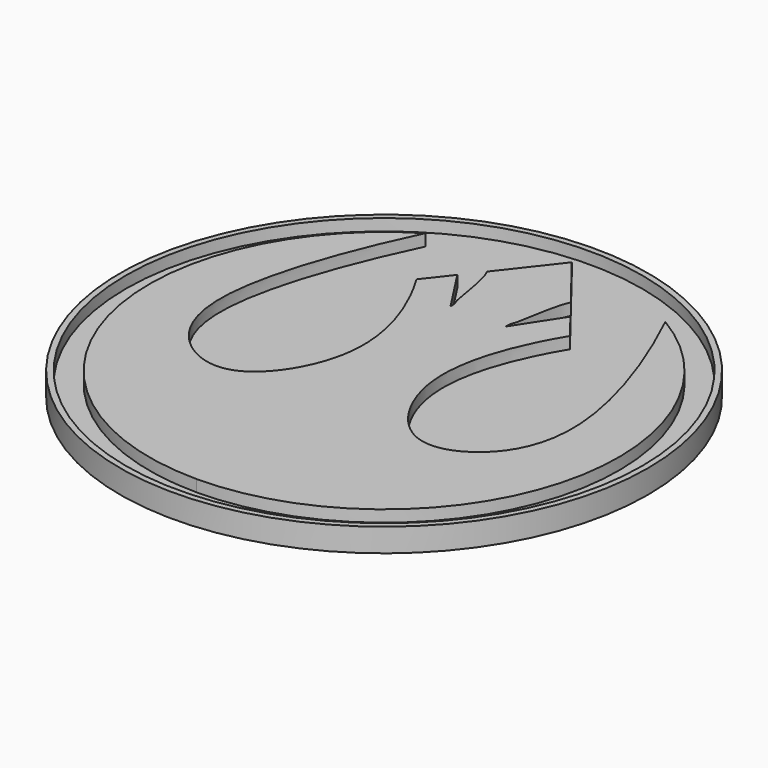
from build123d import *

# Parameters (mm, degrees)
F1_R     = 28.575
F2_DEPTH = 2.54
F0_R     = 27.94
F3_DEPTH = 1.27


with BuildPart() as f2:
    # F1 (on Top) → F2 (new body)
    with BuildSketch(Plane.XY):
        Circle(F1_R)
    extrude(amount=-F2_DEPTH)

    # F0 (on Top) → F3 (cut)
    with BuildSketch(Plane.XY):
        Circle(F0_R)
        with BuildLine():
            ThreePointArc((-12.9824397575, 21.8315427293), (-6.7319690535, 24.491643323), (0, 25.4))
            ThreePointArc((0, 25.4), (6.7319690535, 24.491643323), (12.9824397575, 21.8315427293))
            ThreePointArc((12.9824397575, 21.8315427293), (24.491643323, -6.7319690535), (0, -25.4))
            ThreePointArc((0, -25.4), (-24.491643323, -6.7319690535), (-12.9824397575, 21.8315427293))
        make_face(mode=Mode.SUBTRACT)
        with BuildLine():
            Line((-4.5284444434, 19.6012370521), (0, 25.4))
            ThreePointArc((0, 25.4), (-6.7319690535, 24.491643323), (-12.9824397575, 21.8315427293))
            add(Edge.make_bspline(
                [(-12.9824397575, 21.8315427293), (-16.0030685137, 15.555784787), (-20.8706185969, 2.5324190308), (-17.0205320702, -6.8009951083), (-9.0413114467, -9.8024376533), (-2.0221816541, 1.6054390369), (-6.0604248598, 11.0668484831), (-8.3033278917, 14.767423908)],
                knots=[0, 0, 0, 0, 0.267130235, 0.4415507763, 0.5882558694, 0.7799558658, 1, 1, 1, 1], degree=3))
            Line((-8.3033278917, 14.767423908), (-6.1221701965, 17.5604396079))
            Line((-6.1221701965, 17.5604396079), (-4.5284444434, 19.6012370521))
        make_face()
        with BuildLine():
            ThreePointArc((12.9824397575, 21.8315427293), (6.7319690535, 24.491643323), (0, 25.4))
            Line((0, 25.4), (4.5284444434, 19.6012370521))
            Line((4.5284444434, 19.6012370521), (6.1221701965, 17.5604396079))
            Line((6.1221701965, 17.5604396079), (8.3033278917, 14.767423908))
            add(Edge.make_bspline(
                [(12.9824397575, 21.8315427293), (16.0030685137, 15.555784787), (20.8706185969, 2.5324190308), (17.0205320702, -6.8009951083), (9.0413114467, -9.8024376533), (2.0221816541, 1.6054390369), (6.0604248598, 11.0668484831), (8.3033278917, 14.767423908)],
                knots=[0, 0, 0, 0, 0.267130235, 0.4415507763, 0.5882558694, 0.7799558658, 1, 1, 1, 1], degree=3))
        make_face()
        with BuildLine():
            Line((6.1221701965, 17.5604396079), (4.5284444434, 19.6012370521))
            add(Edge.make_bspline(
                [(4.5284444434, 19.6012370521), (3.7872271779, 18.2003817365), (3.371286388, 13.3642519376), (2.9613813264, 13.5061021755), (2.9711382824, 12.7042779153)],
                knots=[0, 0, 0, 0, 0.6853701695, 1, 1, 1, 1], degree=3))
            Line((2.9711382824, 12.7042779153), (6.1221701965, 17.5604396079))
        make_face()
        with BuildLine():
            add(Edge.make_bspline(
                [(-4.5284444434, 19.6012370521), (-3.7872271779, 18.2003817365), (-3.371286388, 13.3642519376), (-2.9613813264, 13.5061021755), (-2.9711382824, 12.7042779153)],
                knots=[0, 0, 0, 0, 0.6853701695, 1, 1, 1, 1], degree=3))
            Line((-4.5284444434, 19.6012370521), (-6.1221701965, 17.5604396079))
            Line((-6.1221701965, 17.5604396079), (-2.9711382824, 12.7042779153))
        make_face()
    extrude(amount=-F3_DEPTH, mode=Mode.SUBTRACT)


solid = f2.part
